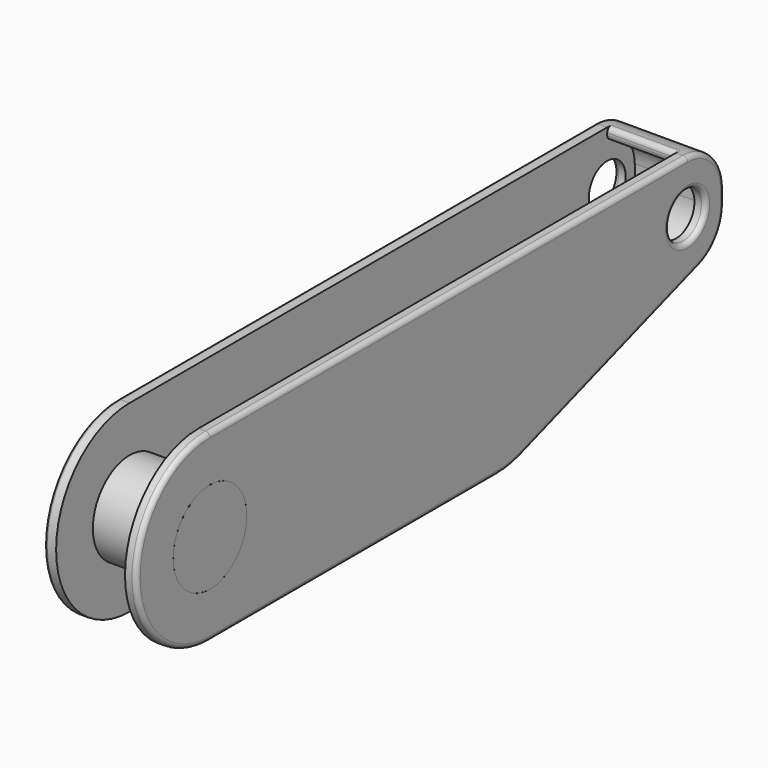
from build123d import *

# Parameters (mm, degrees)
F1_DEPTH  = 6.35
F2_T      = 1.5875
F3_R      = 3.175
F4_DEPTH  = 25.4
F5_R      = 0.635
F6_R      = 0.381
F7_F1_R   = 0.635
F7_F2_R   = 0.635
F7_F3_R   = 0.635
F7_F4_R   = 0.635
F7_F5_R   = 0.635
F9_DEPTH  = 25.4
F10_R     = 6.35
F11_DEPTH = 12.7


# Not quite as in the source:
# - a shell that OpenCascade refuses in one call is made with other operations: the cavity is built on its own and cut out


with BuildPart() as f1:
    # F0 (on Right) → F1 (new body, symmetric)
    with BuildSketch(Plane.YZ):
        with BuildLine():
            ThreePointArc((-38.1, 12.7), (-47.0802561211, 8.9802561211), (-50.8, 0))
            ThreePointArc((-50.8, 0), (-47.0802561211, -8.9802561211), (-38.1, -12.7))
            Line((-38.1, -12.7), (11.6695368579, -12.7))
            ThreePointArc((11.6695368579, -12.7), (13.7589335903, -12.5269478044), (15.7913894262, -12.0125072905))
            Line((15.7913894262, -12.0125072905), (46.5109262841, -1.4717102003))
            ThreePointArc((46.5109262841, -1.4717102003), (49.617658169, 0.8443118739), (50.8, 4.5345434449))
            Line((50.8, 4.5345434449), (50.8, 6.35))
            ThreePointArc((50.8, 6.35), (48.9401280605, 10.8401280605), (44.45, 12.7))
            Line((44.45, 12.7), (-38.1, 12.7))
        make_face()
    extrude(amount=F1_DEPTH, both=True)

    # F2: shell of thickness 1.5875, made by hand


with BuildPart() as f2_core1:
    # F2_t2: copy of F1
    add(f1.part)

    # the walls: a layer under each face that stays
    f2_faces = [f2_core1.faces().sort_by_distance(p)[0] for p in [
        (0, 48.9401280605, 10.8401280605),
        (0, 50.8, 5.4422717225),
        (0, 49.617658169, 0.8443118739),
        (6.35, 0, 0),
        (-6.35, 0, 0),
    ]]
    thicken(f2_faces, amount=-F2_T, mode=Mode.SUBTRACT)


with BuildPart() as f1_1:
    add(f1.part)

    # what is left inside the walls is the cavity
    f2_cavity = [f2_core1.part.solids().sort_by_distance(p)[0] for p in [
        (4.746625, -0.79375, -4.233333),
    ]]
    add(f2_cavity, mode=Mode.SUBTRACT)

    # F3 (on face) → F4 (cut)
    with BuildSketch(Plane(origin=(-6.35, 0, 0), x_dir=(0, -1, 0), z_dir=(-1, 0, 0))):
        with Locations((-44.45, 5.4422717225)):
            Circle(F3_R)
    extrude(amount=-F4_DEPTH, mode=Mode.SUBTRACT)

    # F5
    f5_edges = [f1_1.edges().sort_by_distance(p)[0] for p in [
        (-6.35, 47.625, 5.442272),
        (6.35, 47.625, 5.442272),
    ]]
    fillet(f5_edges, radius=F5_R)

    # F6
    f6_edges = [f1_1.edges().sort_by_distance(p)[0] for p in [
        (-6.35, 48.26, 5.442272),
        (-6.35, 3.175, 12.7),
        (-6.35, 48.940128, 10.840128),
        (-6.35, -50.8, 0),
        (-6.35, 50.8, 5.442272),
        (-6.35, -13.215232, -12.7),
        (-6.35, 49.617658, 0.844312),
        (-6.35, 13.758934, -12.526948),
        (-6.35, 31.151158, -6.742109),
    ]]
    fillet(f6_edges, radius=F6_R)

    # F7: fillet of radius 0.635 on 13 edges, made by hand

    # F7_f1
    f7_f1_edges = [f1_1.edges().sort_by_distance(p)[0] for p in [
        (6.35, 48.9401280605, 10.8401280605),
        (6.35, 50.8, 5.4422717225),
        (6.35, 49.617658169, 0.8443118739),
        (6.35, 3.175, 12.7),
        (6.35, -50.8, 0),
        (6.35, -13.215231571, -12.7),
        (6.35, 13.7589335903, -12.5269478044),
        (6.35, 31.1511578552, -6.7421087454),
    ]]
    fillet(f7_f1_edges, radius=F7_F1_R)

    # F7_f2
    f7_f2_edges = [f1_1.edges().sort_by_distance(p)[0] for p in [
        (0, 46.5109262841, -1.4717102003),
    ]]
    fillet(f7_f2_edges, radius=F7_F2_R)

    # F7_f3
    f7_f3_edges = [f1_1.edges().sort_by_distance(p)[0] for p in [
        (0, 44.45, 11.1125),
    ]]
    fillet(f7_f3_edges, radius=F7_F3_R)

    # F7_f4
    f7_f4_edges = [f1_1.edges().sort_by_distance(p)[0] for p in [
        (0, 45.9956947131, 0.029853211),
    ]]
    fillet(f7_f4_edges, radius=F7_F4_R)

    # F7_f5
    f7_f5_edges = [f1_1.edges().sort_by_distance(p)[0] for p in [
        (0, 44.45, 12.7),
    ]]
    fillet(f7_f5_edges, radius=F7_F5_R)

    # F8 (on face) → F9 (cut)
    with BuildSketch(Plane.YZ.offset(6.35)):
        with BuildLine():
            ThreePointArc((-31.75, 0), (-33.6098719395, 4.4901280605), (-38.1, 6.35))
            Line((-38.1, 6.35), (-38.1, -6.35))
            ThreePointArc((-38.1, -6.35), (-33.6098719395, -4.4901280605), (-31.75, 0))
        make_face()
        with BuildLine():
            Line((-38.1, -6.35), (-38.1, 6.35))
            ThreePointArc((-38.1, 6.35), (-44.45, 0), (-38.1, -6.35))
        make_face()
    extrude(amount=-F9_DEPTH, mode=Mode.SUBTRACT)


with BuildPart() as f11:
    # F10 (on face) → F11 (new body)
    with BuildSketch(Plane.YZ.offset(6.35)):
        with Locations((-38.1, 0)):
            Circle(F10_R)
    extrude(amount=-F11_DEPTH)


solid = Compound([f1_1.part, f11.part])
